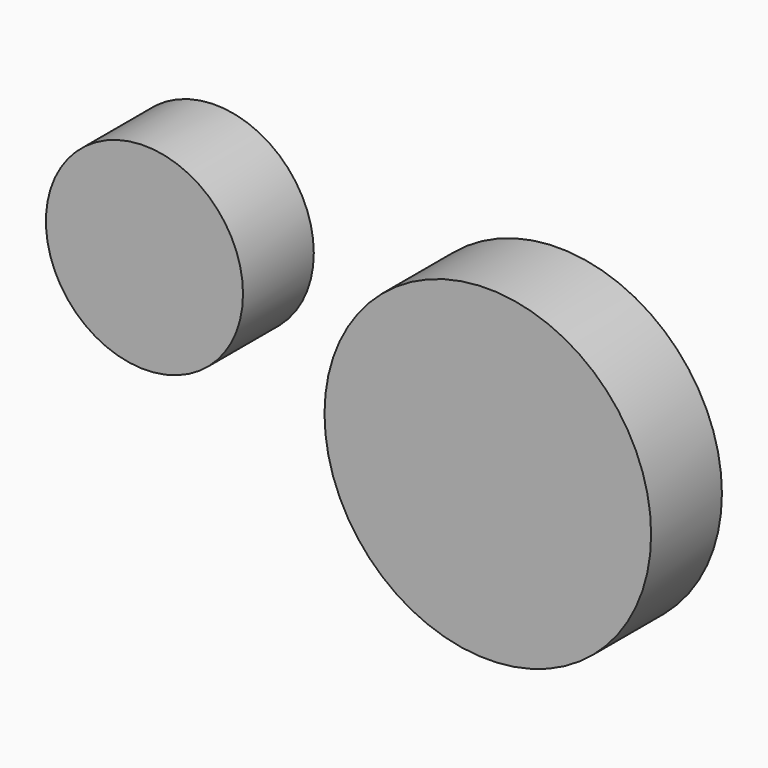
from build123d import *

# Parameters (mm, degrees)
F1_R     = 24.2731402163
F1_R_2   = 7.8379343963
F2_DEPTH = 25.4
F0_R     = 46.8778023243
F4_DEPTH = 25.4
F5_R     = 28.2899115296
F5_R_2   = 20.4147682213
F5_R_3   = 10.0236326285
F6_DEPTH = 25.4


# Not quite as in the source:
# - the program builds the solid bodies; features that only make, move or delete a surface that nothing else refers to are left out


with BuildPart() as f2:
    # F1 (on Front) → F2 (new body)
    with BuildSketch(Plane.XZ):
        Circle(F1_R)
        Circle(F1_R_2, mode=Mode.SUBTRACT)
    extrude(amount=F2_DEPTH)

    # F0 (on Front) → F4 (join)
    with BuildSketch(Plane.XZ):
        Circle(F0_R)
    extrude(amount=F4_DEPTH)


with BuildPart() as f6:
    # F5 (on Front) → F6 (new body)
    with BuildSketch(Plane.XZ):
        with Locations((-98.5608547926, 22.6546935737)):
            Circle(F5_R)
        with Locations((-98.5608547926, 22.6546935737)):
            Circle(F5_R_2, mode=Mode.SUBTRACT)
        with Locations((-98.5608547926, 22.6546935737)):
            Circle(F5_R_2)
        with Locations((-98.5608547926, 22.6546935737)):
            Circle(F5_R_3, mode=Mode.SUBTRACT)
        with Locations((-98.5608547926, 22.6546935737)):
            Circle(F5_R_3)
    extrude(amount=F6_DEPTH)


solid = Compound([f2.part, f6.part])
